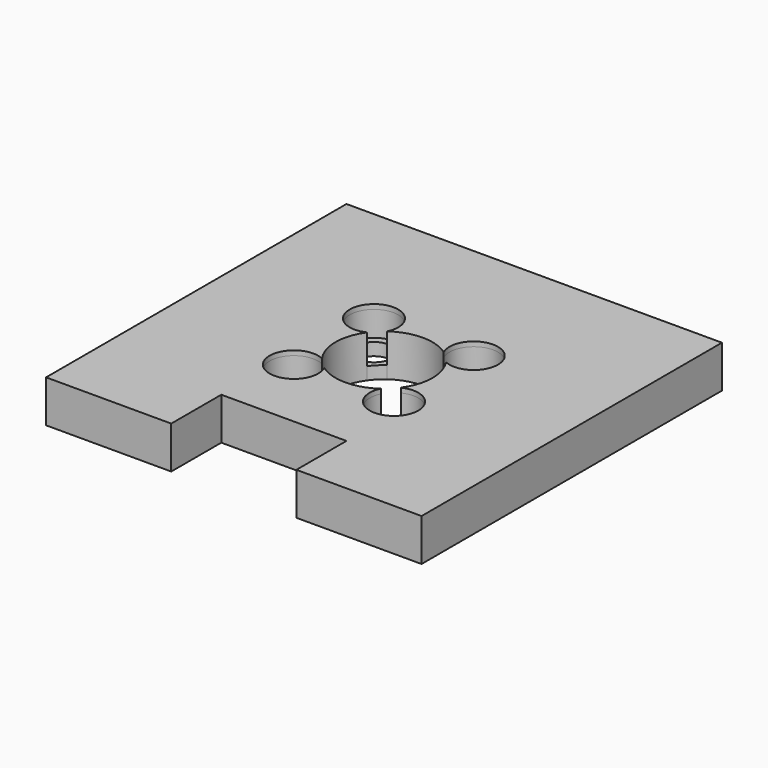
from build123d import *
from build123d import SkipClean  # not in build123d's __all__

# Parameters (mm, degrees)
F1_DEPTH = 3.429
F0_R     = 1.397
F2_DEPTH = 3.048
F3_DEPTH = 2.032


with BuildPart() as f1:
    # F0 (on Top) → F1 (new body)
    with BuildSketch(Plane.XY):
        Polygon((15.24, -15.24), (15.24, 15.24), (-15.24, 15.24), (-15.24, -15.24), (-5.08, -15.24), (-5.08, -10.16), (5.08, -10.16), (5.08, -15.24), align=None)
        with BuildLine():
            ThreePointArc((3.2465476869, 2.227082647), (3.760427319, 1.1658281942), (3.937, 0))
            ThreePointArc((3.937, 0), (3.7477069339, -1.2060935857), (3.1980303594, -2.2962079219))
            ThreePointArc((3.1980303594, -2.2962079219), (5.1057127753, -2.3937225549), (6.0325, -4.064))
            ThreePointArc((6.0325, -4.064), (3.6195376595, -5.9816666754), (2.2962079219, -3.1980303594))
            ThreePointArc((2.2962079219, -3.1980303594), (0, -3.937), (-2.2962079219, -3.1980303594))
            ThreePointArc((-2.2962079219, -3.1980303594), (-2.1463333246, -3.6195376595), (-2.0955, -4.064))
            ThreePointArc((-2.0955, -4.064), (-5.7342774451, -5.1057127753), (-3.1980303594, -2.2962079219))
            ThreePointArc((-3.1980303594, -2.2962079219), (-3.937, 0), (-3.1980303594, 2.2962079219))
            ThreePointArc((-3.1980303594, 2.2962079219), (-5.7342774451, 5.1057127753), (-2.0955, 4.064))
            ThreePointArc((-2.0955, 4.064), (-2.1463333246, 3.6195376595), (-2.2962079219, 3.1980303594))
            ThreePointArc((-2.2962079219, 3.1980303594), (-0.0131703869, 3.9369779706), (2.2747600024, 3.2133216352))
            ThreePointArc((2.2747600024, 3.2133216352), (3.664202861, 5.9391021751), (6.0417570924, 4.0135718882))
            ThreePointArc((6.0417570924, 4.0135718882), (5.1333549146, 2.3549022836), (3.2465476869, 2.227082647))
        make_face(mode=Mode.SUBTRACT)
    extrude(amount=F1_DEPTH)

    # F0 (on Top) → F2 (join)
    with BuildSketch(Plane.XY):
        with BuildLine():
            ThreePointArc((-3.1980303594, 2.2962079219), (-2.7838793975, 2.7838793975), (-2.2962079219, 3.1980303594))
            ThreePointArc((-2.2962079219, 3.1980303594), (-2.1463333246, 3.6195376595), (-2.0955, 4.064))
            ThreePointArc((-2.0955, 4.064), (-5.7342774451, 5.1057127753), (-3.1980303594, 2.2962079219))
        make_face()
        with Locations((-4.064, 4.064)):
            Circle(F0_R, mode=Mode.SUBTRACT)
        with BuildLine():
            ThreePointArc((2.2747600024, 3.2133216352), (2.8043495655, 2.763257591), (3.2465476869, 2.227082647))
            ThreePointArc((3.2465476869, 2.227082647), (5.1333549146, 2.3549022836), (6.0417570924, 4.0135718882))
            ThreePointArc((6.0417570924, 4.0135718882), (3.664202861, 5.9391021751), (2.2747600024, 3.2133216352))
        make_face()
        with Locations((4.064, 4.064)):
            Circle(F0_R, mode=Mode.SUBTRACT)
        with BuildLine():
            ThreePointArc((-2.0955, -4.064), (-2.1463333246, -3.6195376595), (-2.2962079219, -3.1980303594))
            ThreePointArc((-2.2962079219, -3.1980303594), (-2.7838793975, -2.7838793975), (-3.1980303594, -2.2962079219))
            ThreePointArc((-3.1980303594, -2.2962079219), (-5.7342774451, -5.1057127753), (-2.0955, -4.064))
        make_face()
        with Locations((-4.064, -4.064)):
            Circle(F0_R, mode=Mode.SUBTRACT)
        with BuildLine():
            ThreePointArc((6.0325, -4.064), (5.1057127753, -2.3937225549), (3.1980303594, -2.2962079219))
            ThreePointArc((3.1980303594, -2.2962079219), (2.7838793975, -2.7838793975), (2.2962079219, -3.1980303594))
            ThreePointArc((2.2962079219, -3.1980303594), (3.6195376595, -5.9816666754), (6.0325, -4.064))
        make_face()
        with Locations((4.064, -4.064)):
            Circle(F0_R, mode=Mode.SUBTRACT)
    extrude(amount=F2_DEPTH)

    # F3 (cut): faces of the model
    f3_faces = [f1.faces().sort_by_distance(p)[0] for p in [
        (-2.8232493975, 2.8232493975, 3.048),
        (-5.4165696988, -5.4165696988, 3.048),
        (2.8440090574, 2.8023359547, 3.048),
        (5.4165696988, -5.4165696988, 3.048),
    ]]
    with SkipClean():  # cleaning this boolean's faces spoils the solid; the shape is the same uncleaned
        extrude(f3_faces, amount=-F3_DEPTH, mode=Mode.SUBTRACT)


solid = f1.part
